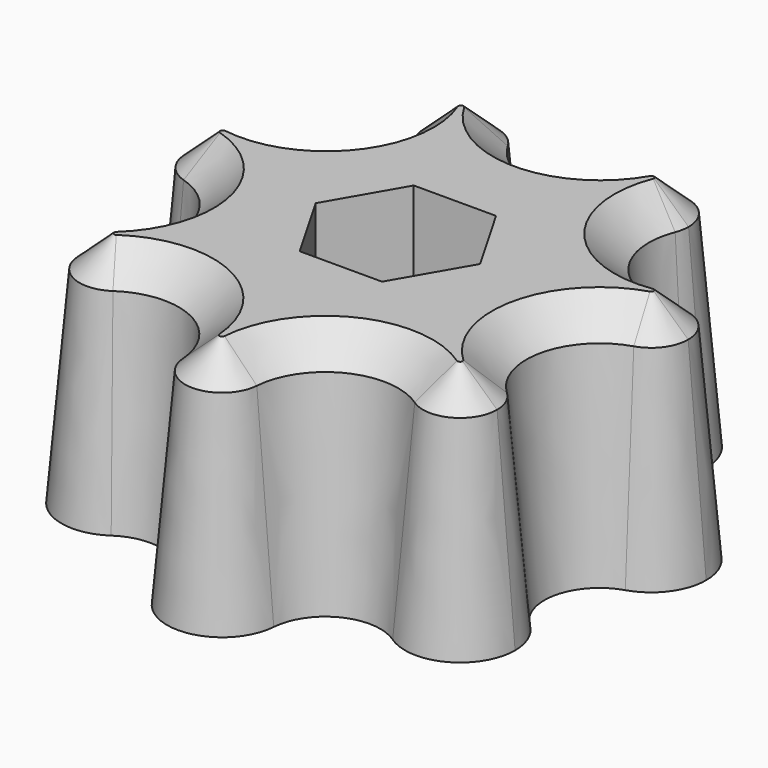
from build123d import *

# Parameters (mm, degrees)
F0_R                   = 9.525
F1_DEPTH               = 19.05
DRAFT_F1_DRAFTED_ANGLE = 5
F2_DEPTH               = 19.05
F3_SIZE                = 2.54
F4_R                   = 6.845
F4_R_2                 = 4.445
F5_DEPTH               = 3.175
F5_DEPTH_BACK          = 1.2


# Not quite as in the source:
# - an extrude with a draft is written as a straight extrude whose walls are then drafted


with BuildPart() as f1:
    # F0 (on Top) → F1 (new body)
    with BuildSketch(Plane.XY):
        with BuildLine():
            ThreePointArc((-11.7537259014, 14.2624427644), (-6.8244127775, 11.5381076989), (-3.2311559552, 15.875))
            ThreePointArc((-3.2311559552, 15.875), (-3.3815539442, 17.0173861435), (-3.8224985368, 18.0819205592))
            ThreePointArc((-3.8224985368, 18.0819205592), (-9.5600909619, 19.8517334355), (-11.7537259014, 14.2624427644))
        make_face()
        with BuildLine():
            ThreePointArc((-3.8224985368, 18.0819205592), (-3.3815539442, 17.0173861435), (-3.2311559552, 15.875))
            ThreePointArc((-3.2311559552, 15.875), (-6.8244127775, 11.5381076989), (-11.7537259014, 14.2624427644))
            ThreePointArc((-11.7537259014, 14.2624427644), (-12.4115747842, 9.8979006045), (-16.520303612, 8.2853433689))
            ThreePointArc((-16.520303612, 8.2853433689), (-13.8325857366, 6.7998942059), (-12.7643113764, 3.920801209))
            ThreePointArc((-12.7643113764, 3.920801209), (-14.5571245428, 0.3694344449), (-18.4791550035, -0.2969453328))
            ThreePointArc((-18.4791550035, -0.2969453328), (-15.4769806059, -3.5325198266), (-16.7779831146, -7.7502663683))
            ThreePointArc((-16.7779831146, -7.7502663683), (-12.0107488571, -6.9402806896), (-9.3619675986, -10.9858408621))
            ThreePointArc((-9.3619675986, -10.9858408621), (-9.8734638397, -13.0482903469), (-11.2894034819, -14.6327275378))
            ThreePointArc((-11.2894034819, -14.6327275378), (-6.8879043585, -14.302880778), (-4.4014991234, -17.9497674536))
            ThreePointArc((-4.4014991234, -17.9497674536), (-0.1650387908, -13.2091661534), (4.4138411184, -17.6199206938))
            ThreePointArc((4.4138411184, -17.6199206938), (4.4107545404, -17.7849594845), (4.4014991234, -17.9497674536))
            ThreePointArc((4.4014991234, -17.9497674536), (6.8879043585, -14.302880778), (11.2894034819, -14.6327275378))
            ThreePointArc((11.2894034819, -14.6327275378), (10.324928772, -8.2338559378), (16.7779831146, -7.7502663683))
            ThreePointArc((16.7779831146, -7.7502663683), (15.4769806059, -3.5325198266), (18.4791550035, -0.2969453328))
            ThreePointArc((18.4791550035, -0.2969453328), (12.8749755885, 2.938629161), (16.520303612, 8.2853433689))
            ThreePointArc((16.520303612, 8.2853433689), (12.4115747842, 9.8979006045), (11.7537259014, 14.2624427644))
            ThreePointArc((11.7537259014, 14.2624427644), (5.7299031853, 11.8982665645), (3.8224985368, 18.0819205592))
            ThreePointArc((3.8224985368, 18.0819205592), (0, 15.875), (-3.8224985368, 18.0819205592))
        make_face()
        Circle(F0_R, mode=Mode.SUBTRACT)
        with BuildLine():
            ThreePointArc((12.0588381919, 15.875), (8.7873832171, 20.1384431294), (3.8224985368, 18.0819205592))
            ThreePointArc((3.8224985368, 18.0819205592), (5.7299031853, 11.8982665645), (11.7537259014, 14.2624427644))
            ThreePointArc((11.7537259014, 14.2624427644), (11.9818893747, 15.0544157039), (12.0588381919, 15.875))
        make_face()
        with BuildLine():
            ThreePointArc((-12.7643113764, 3.920801209), (-13.8325857366, 6.7998942059), (-16.520303612, 8.2853433689))
            ThreePointArc((-16.520303612, 8.2853433689), (-21.481329401, 4.902973257), (-18.4791550035, -0.2969453328))
            ThreePointArc((-18.4791550035, -0.2969453328), (-14.5571245428, 0.3694344449), (-12.7643113764, 3.920801209))
        make_face()
        with BuildLine():
            ThreePointArc((21.5919936132, 3.920801209), (20.0572454917, 7.2663679672), (16.520303612, 8.2853433689))
            ThreePointArc((16.520303612, 8.2853433689), (12.8749755885, 2.938629161), (18.4791550035, -0.2969453328))
            ThreePointArc((18.4791550035, -0.2969453328), (20.7295192589, 1.299773257), (21.5919936132, 3.920801209))
        make_face()
        with BuildLine():
            ThreePointArc((-9.3619675986, -10.9858408621), (-12.0107488571, -6.9402806896), (-16.7779831146, -7.7502663683))
            ThreePointArc((-16.7779831146, -7.7502663683), (-17.2266886619, -13.7378257865), (-11.2894034819, -14.6327275378))
            ThreePointArc((-11.2894034819, -14.6327275378), (-9.8734638397, -13.0482903469), (-9.3619675986, -10.9858408621))
        make_face()
        with BuildLine():
            ThreePointArc((18.1896498354, -10.9858408621), (17.8213688895, -9.2207810023), (16.7779831146, -7.7502663683))
            ThreePointArc((16.7779831146, -7.7502663683), (10.324928772, -8.2338559378), (11.2894034819, -14.6327275378))
            ThreePointArc((11.2894034819, -14.6327275378), (15.8382582018, -14.8881857394), (18.1896498354, -10.9858408621))
        make_face()
        with BuildLine():
            ThreePointArc((4.4138411184, -17.6199206938), (-0.1650387908, -13.2091661534), (-4.4014991234, -17.9497674536))
            ThreePointArc((-4.4014991234, -17.9497674536), (0, -22.0337618122), (4.4014991234, -17.9497674536))
            ThreePointArc((4.4014991234, -17.9497674536), (4.4107545404, -17.7849594845), (4.4138411184, -17.6199206938))
        make_face()
        Circle(F0_R)
        Polygon((-6.5991135768, 0), (-3.2995567884, 5.715), (3.2995567884, 5.715), (6.5991135768, 0), (3.2995567884, -5.715), (-3.2995567884, -5.715), align=None, mode=Mode.SUBTRACT)
    extrude(amount=F1_DEPTH)

    # draft_F1_drafted
    draft_f1_drafted_walls = [f1.faces().sort_by_distance(p)[0] for p in [
        (-9.5600909619, 19.8517334355, 12.7),
        (-12.4115747842, 9.8979006045, 12.7),
        (-21.481329401, 4.902973257, 12.7),
        (-15.4769806059, -3.5325198266, 12.7),
        (-17.2266886619, -13.7378257865, 12.7),
        (-6.8879043585, -14.302880778, 12.7),
        (0, -22.0337618122, 12.7),
        (6.8879043585, -14.302880778, 12.7),
        (17.2266886619, -13.7378257865, 12.7),
        (15.4769806059, -3.5325198266, 12.7),
        (21.481329401, 4.902973257, 12.7),
        (12.4115747842, 9.8979006045, 12.7),
        (9.5600909619, 19.8517334355, 12.7),
        (0, 15.875, 12.7),
        (-4.9493351826, -2.8575, 12.7),
        (-4.9493351826, 2.8575, 12.7),
        (0, 5.715, 12.7),
        (4.9493351826, 2.8575, 12.7),
        (4.9493351826, -2.8575, 12.7),
        (0, -5.715, 12.7),
    ]]
    draft(draft_f1_drafted_walls, neutral_plane=Plane.XY, angle=DRAFT_F1_DRAFTED_ANGLE)

    # F0 (on Top) → F2 (join, through all)
    with BuildSketch(Plane.XY):
        Circle(F0_R)
        Polygon((-6.5991135768, 0), (-3.2995567884, 5.715), (3.2995567884, 5.715), (6.5991135768, 0), (3.2995567884, -5.715), (-3.2995567884, -5.715), align=None, mode=Mode.SUBTRACT)
    extrude(amount=F2_DEPTH)

    # F3
    f3_edges = [f1.edges().sort_by_distance(p)[0] for p in [
        (-8.836955, 18.350126, 19.05),
        (0, 14.208341, 19.05),
        (-11.108528, 8.858756, 19.05),
        (-19.856457, 4.532107, 19.05),
        (-13.852108, -3.161653, 19.05),
        (-15.923642, -12.698681, 19.05),
        (-6.164768, -12.801273, 19.05),
        (0, -20.367103, 19.05),
        (6.164768, -12.801273, 19.05),
        (15.923642, -12.698681, 19.05),
        (13.852108, -3.161653, 19.05),
        (19.856457, 4.532107, 19.05),
        (11.108528, 8.858756, 19.05),
        (8.836955, 18.350126, 19.05),
    ]]
    chamfer(f3_edges, length=F3_SIZE)

    # F4 (on face) → F5 (join, two sides)
    with BuildSketch(Plane(origin=(0, 0, 0), x_dir=(1, 0, 0), z_dir=(0, 0, -1))) as f5_sk:
        Circle(F4_R)
        Circle(F4_R_2, mode=Mode.SUBTRACT)
    extrude(amount=F5_DEPTH)
    extrude(f5_sk.sketch, amount=-F5_DEPTH_BACK)


solid = f1.part
